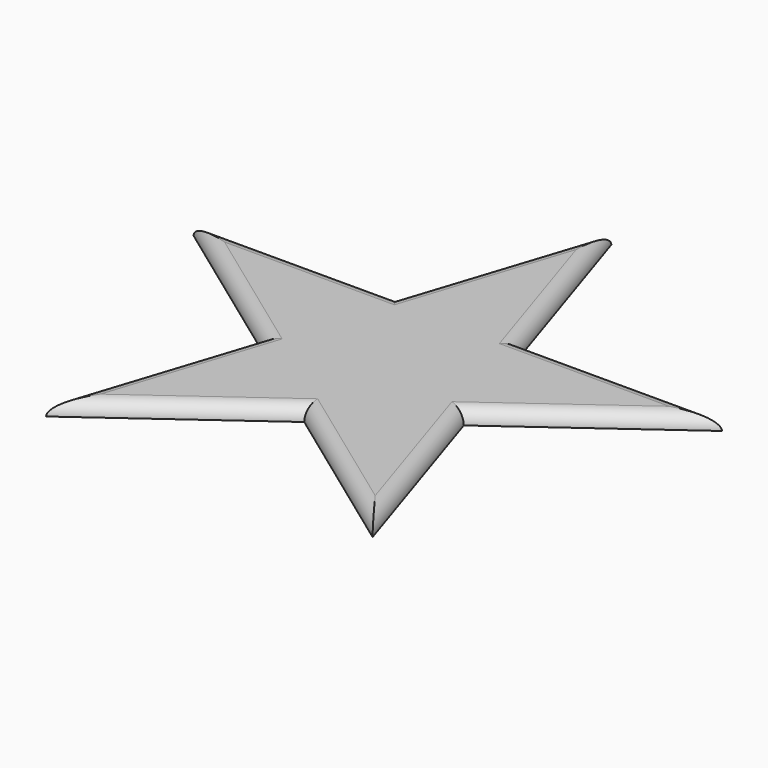
from build123d import *

# Parameters (mm, degrees)
F1_DEPTH = 2.5
F2_R     = 2.49999


# Not quite as in the source:
# - a fillet or chamfer is up to 0.001 mm smaller than in the source, because OpenCascade refuses the exact size


with BuildPart() as f1:
    # F0 (on Top) → F1 (new body)
    with BuildSketch(Plane.XY):
        Polygon((-11.4502134028, 15.7598667131), (-48.5038823311, 15.7598667131), (-18.5268344641, -6.0197334262), (-29.9770478669, -41.2598667131), (0, -19.4802665738), (29.9770478669, -41.2598667131), (18.5268344641, -6.0197334262), (48.5038823311, 15.7598667131), (11.4502134028, 15.7598667131), (0, 51), align=None)
    extrude(amount=F1_DEPTH)

    # F2 (radius 2.5 in the source; OpenCascade refuses exactly that, so slightly less here)
    f2_edges = [f1.edges().sort_by_distance(p)[0] for p in [
        (-5.725107, 33.379933, 2.5),
        (-29.977048, 15.759867, 2.5),
        (-33.515358, 4.870067, 2.5),
        (-24.251941, -23.6398, 2.5),
        (14.988524, -30.370067, 2.5),
        (24.251941, -23.6398, 2.5),
        (33.515358, 4.870067, 2.5),
        (29.977048, 15.759867, 2.5),
        (5.725107, 33.379933, 2.5),
        (-14.988524, -30.370067, 2.5),
    ]]
    fillet(f2_edges, radius=F2_R)


solid = f1.part
